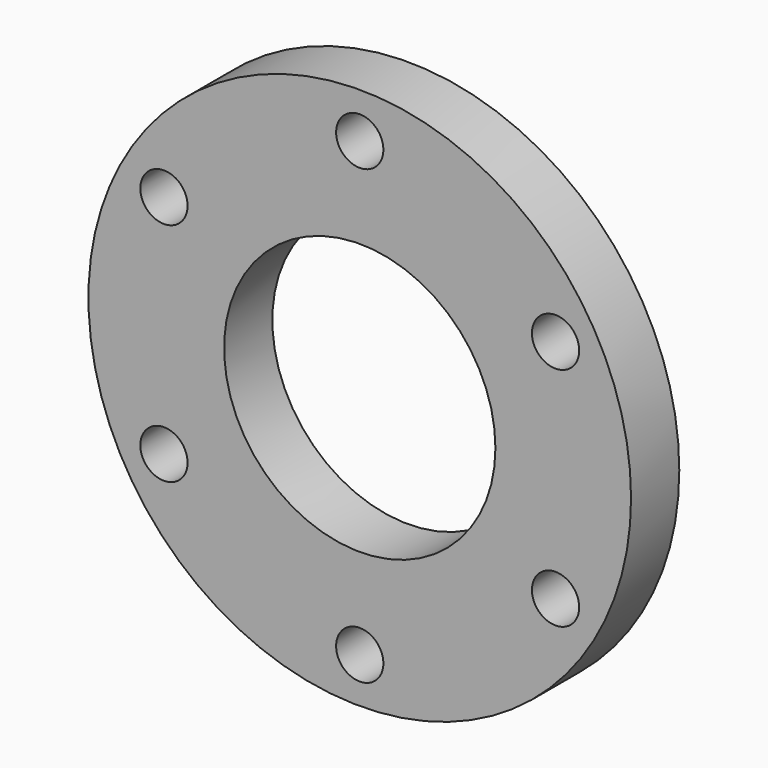
from build123d import *

# Parameters (mm, degrees)
F0_R            = 28.575
F0_R_2          = 14.2875
F1_DEPTH        = 6.35
F2_R            = 2.4892
F3_DEPTH        = 6.351
F3_COPIES_COUNT = 6


# Not quite as in the source:
# - a pattern or mirror of a feature is missing from the dataset's text; its kind, count and spacing are read off the source's solid


with BuildPart() as f1:
    # F0 (on Front) → F1 (new body)
    with BuildSketch(Plane.XZ):
        Circle(F0_R)
        Circle(F0_R_2, mode=Mode.SUBTRACT)
    extrude(amount=F1_DEPTH)

    # F2 (on face) → F3 (cut, through all)
    with BuildSketch(Plane.XZ.offset(6.35)):
        with Locations((0, 23.8125)):
            Circle(F2_R)
    f3 = extrude(amount=-F3_DEPTH, mode=Mode.SUBTRACT)

    # F3_copies: F3 ×6 about axis
    f3_copies_axis = Axis((0, 0, 0), (0, 1, 0))
    for i in range(1, F3_COPIES_COUNT):
        add(f3.rotate(f3_copies_axis, i * 360 / F3_COPIES_COUNT), mode=Mode.SUBTRACT)


solid = f1.part
